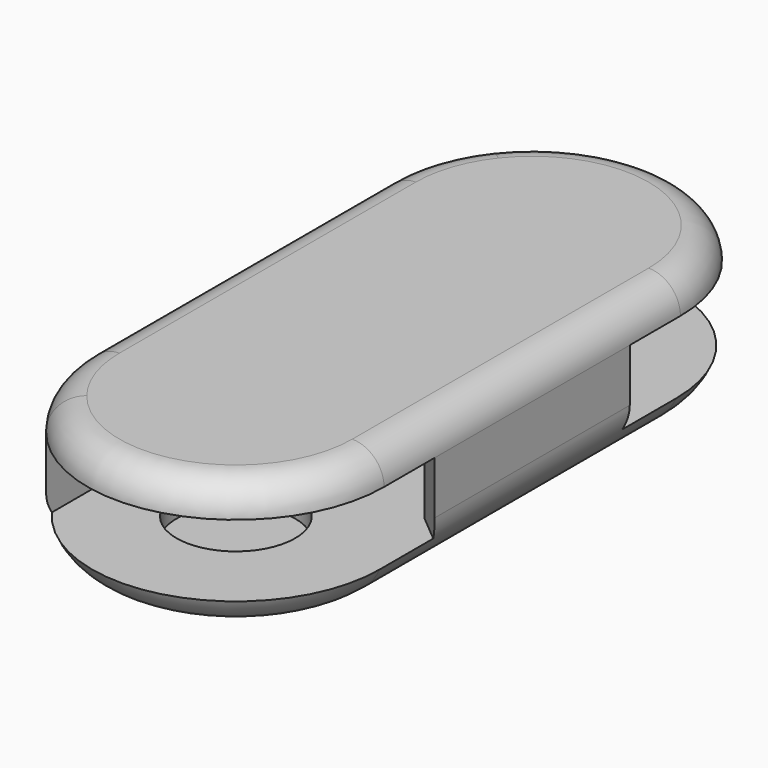
from build123d import *

# Parameters (mm, degrees)
F1_DEPTH    = 3
F2_R        = 5.6
F3_DEPTH    = 2
F5_DEPTH    = 10
F7_DEPTH    = 3
F8_R        = 2.99999
F9_T1_DEPTH = 35
F9_T4_ANGLE = 180
F9_T6_ANGLE = 180


# Not quite as in the source:
# - a fillet or chamfer that OpenCascade refuses, or shapes differently, is made with other operations: its cross-section is extruded or revolved along the edge and cut away or added
# - a fillet or chamfer is up to 0.001 mm smaller than in the source, because OpenCascade refuses the exact size


with BuildPart() as f1:
    # F0 (on Top) → F1 (new body)
    with BuildSketch(Plane.XY):
        with BuildLine():
            Line((14, -17.5), (14, 17.5))
            ThreePointArc((14, 17.5), (0, 31.5), (-14, 17.5))
            Line((-14, 17.5), (-14, -17.5))
            ThreePointArc((-14, -17.5), (0, -31.5), (14, -17.5))
        make_face()
    extrude(amount=F1_DEPTH)

    # F2 (on face) → F3 (cut)
    with BuildSketch(Plane.XY.offset(3)):
        with Locations((0, 17.5)):
            Circle(F2_R)
        with Locations((0, -17.5)):
            Circle(F2_R)
    extrude(amount=-F3_DEPTH, mode=Mode.SUBTRACT)

    # F4 (on Top) → F5 (join)
    with BuildSketch(Plane.XY):
        with BuildLine():
            Line((-11, -26.1602540378), (-11, 26.1602540378))
            ThreePointArc((-11, 26.1602540378), (-13.2287565553, 22.082575695), (-14, 17.5))
            Line((-14, 17.5), (-14, -17.5))
            ThreePointArc((-14, -17.5), (-13.2287565553, -22.082575695), (-11, -26.1602540378))
        make_face()
        Polygon((14, -11.5172988935), (14, 11.5172988935), (11, 9), (11, -9), align=None)
    extrude(amount=F5_DEPTH)

    # F6 (on face) → F7 (join)
    with BuildSketch(Plane.XY.offset(10)):
        with BuildLine():
            Line((14, -17.5), (14, 17.5))
            ThreePointArc((14, 17.5), (4.582575695, 30.7287565553), (-11, 26.1602540378))
            Line((-11, 26.1602540378), (-11, -26.1602540378))
            ThreePointArc((-11, -26.1602540378), (4.582575695, -30.7287565553), (14, -17.5))
        make_face()
        with BuildLine():
            Line((-11, -26.1602540378), (-11, 26.1602540378))
            ThreePointArc((-11, 26.1602540378), (-13.2287565553, 22.082575695), (-14, 17.5))
            Line((-14, 17.5), (-14, -17.5))
            ThreePointArc((-14, -17.5), (-13.2287565553, -22.082575695), (-11, -26.1602540378))
        make_face()
    extrude(amount=F7_DEPTH)

    # F8 (radius 3 in the source; OpenCascade refuses exactly that, so slightly less here)
    f8_edges = [f1.edges().sort_by_distance(p)[0] for p in [
        (14, 0, 13),
        (0, 31.5, 13),
        (-14, 0, 13),
        (0, -31.5, 13),
    ]]
    fillet(f8_edges, radius=F8_R)

    # F9: fillet of radius 5 on 4 edges, made by hand

    # F9_s2 → F9_t1 (cut)
    with BuildSketch(Plane.XZ.offset(-17.5)):
        with BuildLine():
            ThreePointArc((14, 5), (12.5355339059, 1.4644660941), (9, 0))
            Line((9, 0), (14, 0))
            Line((14, 0), (14, 5))
        make_face()
        with BuildLine():
            ThreePointArc((-9, 0), (-12.5355339059, 1.4644660941), (-14, 5))
            Line((-14, 5), (-14, 0))
            Line((-14, 0), (-9, 0))
        make_face()
    extrude(amount=F9_T1_DEPTH, mode=Mode.SUBTRACT)

    # F9_s3 → F9_t4 (revolve, cut)
    with BuildSketch(Plane.XZ.offset(17.5)):
        with BuildLine():
            ThreePointArc((14, 5), (12.5355339059, 1.4644660941), (9, 0))
            Line((9, 0), (14, 0))
            Line((14, 0), (14, 5))
        make_face()
    revolve(axis=Axis((0, -17.5, 0), (0, 0, -1)), revolution_arc=F9_T4_ANGLE, mode=Mode.SUBTRACT)

    # F9_s5 → F9_t6 (revolve, cut)
    with BuildSketch(Plane.XZ.offset(-17.5)):
        with BuildLine():
            ThreePointArc((-14, 5), (-12.5355339059, 1.4644660941), (-9, 0))
            Line((-9, 0), (-14, 0))
            Line((-14, 0), (-14, 5))
        make_face()
    revolve(axis=Axis((0, 17.5, 0), (0, 0, -1)), revolution_arc=F9_T6_ANGLE, mode=Mode.SUBTRACT)


solid = f1.part
